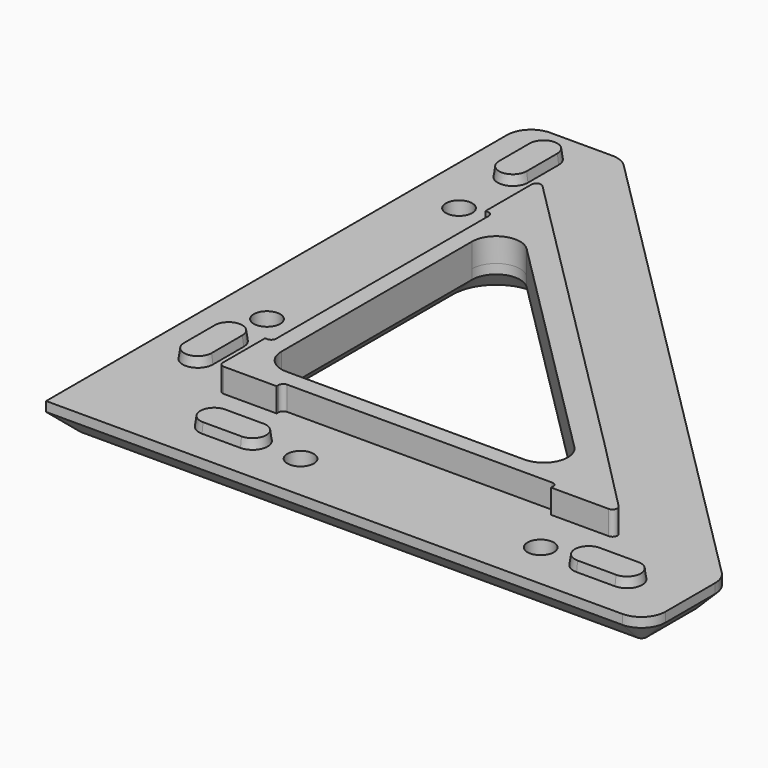
from build123d import *

# Parameters (mm, degrees)
F1_DEPTH  = 6
F2_R      = 5
F4_DEPTH  = 5
F5_SIZE   = 4
F6_R      = 1
F8_D      = 5.5
F9_W      = 57.1730165467
F9_H      = 1.5
F9_W_2    = 1.5
F9_H_2    = 57.372583002
F10_DEPTH = 5
F11_R     = 1
F13_DEPTH = 2
F13_TAPER = 8


with BuildPart() as f1:
    # F0 (on Top) → F1 (new body)
    with BuildSketch(Plane.XY):
        Polygon((20, 125), (0, 125), (0, 0), (125, 0), (125, 20), align=None)
        Polygon((25, 25), (25, 91.7157287525), (91.7157287525, 25), align=None, mode=Mode.SUBTRACT)
    extrude(amount=F1_DEPTH)

    # F2
    f2_edges = [f1.edges().sort_by_distance(p)[0] for p in [
        (25, 91.715729, 3),
        (91.715729, 25, 3),
        (25, 25, 3),
        (0, 125, 3),
        (20, 125, 3),
        (125, 20, 3),
        (125, 0, 3),
    ]]
    fillet(f2_edges, radius=F2_R)

    # F3 (on face) → F4 (join)
    with BuildSketch(Plane.XY.offset(6)):
        Polygon((86.7157287525, 37.0710678119), (37.0710678119, 86.7157287525), (20, 103.7867965644), (20, 79.6446609407), (20, 30), (20, 20), (30, 20), (79.6446609407, 20), (103.5650894046, 20), align=None)
        with BuildLine():
            ThreePointArc((30, 25), (26.4644660941, 26.4644660941), (25, 30))
            Line((25, 30), (25, 79.6446609407))
            ThreePointArc((25, 79.6446609407), (28.0865828382, 84.2640586032), (33.5355339059, 83.1801948466))
            Line((33.5355339059, 83.1801948466), (83.1801948466, 33.5355339059))
            ThreePointArc((83.1801948466, 33.5355339059), (84.2640586032, 28.0865828382), (79.6446609407, 25))
            Line((79.6446609407, 25), (30, 25))
        make_face(mode=Mode.SUBTRACT)
    extrude(amount=F4_DEPTH)

    # F5
    f5_edges = [f1.edges().sort_by_distance(p)[0] for p in [
        (58.357864, 58.357864, 0),
        (72.5, 72.5, 0),
    ]]
    chamfer(f5_edges, length=F5_SIZE)

    # F6
    f6_edges = [f1.edges().sort_by_distance(p)[0] for p in [
        (20, 103.786797, 8.5),
        (20, 20, 8.5),
        (103.565089, 20, 8.5),
    ]]
    fillet(f6_edges, radius=F6_R)

    # F8 (through all)
    with Locations(Plane(origin=(0, 0, 0), x_dir=(1, 0, 0), z_dir=(0, 0, -1))):
        with Locations((95, -10), (45, -10), (10, -45), (10, -95)):
            Hole(F8_D / 2)

    # F9 (on face) → F10 (cut, through all)
    with BuildSketch(Plane.XY.offset(11)):
        with Locations((60.5865082733, 20.75)):
            Rectangle(F9_W, F9_H)
        with Locations((20.75, 60.686291501)):
            Rectangle(F9_W_2, F9_H_2)
    extrude(amount=-F10_DEPTH, mode=Mode.SUBTRACT)

    # F11
    f11_edges = [f1.edges().sort_by_distance(p)[0] for p in [
        (21.5, 89.372583, 8.5),
        (21.5, 32, 8.5),
        (32, 21.5, 8.5),
        (89.173017, 21.5, 8.5),
    ]]
    fillet(f11_edges, radius=F11_R)

    # F12 (on face) → F13 (join)
    with BuildSketch(Plane.XY.offset(6)):
        with BuildLine():
            Line((6.85, 117), (6.85, 109))
            ThreePointArc((6.85, 109), (10, 105.85), (13.15, 109))
            Line((13.15, 109), (13.15, 117))
            ThreePointArc((13.15, 117), (10, 120.15), (6.85, 117))
        make_face()
        with BuildLine():
            Line((6.85, 35), (6.85, 27))
            ThreePointArc((6.85, 27), (10, 23.85), (13.15, 27))
            Line((13.15, 27), (13.15, 35))
            ThreePointArc((13.15, 35), (10, 38.15), (6.85, 35))
        make_face()
        with BuildLine():
            Line((35, 13.15), (27, 13.15))
            ThreePointArc((27, 13.15), (23.85, 10), (27, 6.85))
            Line((27, 6.85), (35, 6.85))
            ThreePointArc((35, 6.85), (38.15, 10), (35, 13.15))
        make_face()
        with BuildLine():
            Line((113, 13.15), (105, 13.15))
            ThreePointArc((105, 13.15), (101.85, 10), (105, 6.85))
            Line((105, 6.85), (113, 6.85))
            ThreePointArc((113, 6.85), (116.15, 10), (113, 13.15))
        make_face()
    extrude(amount=F13_DEPTH, taper=F13_TAPER)


solid = f1.part
